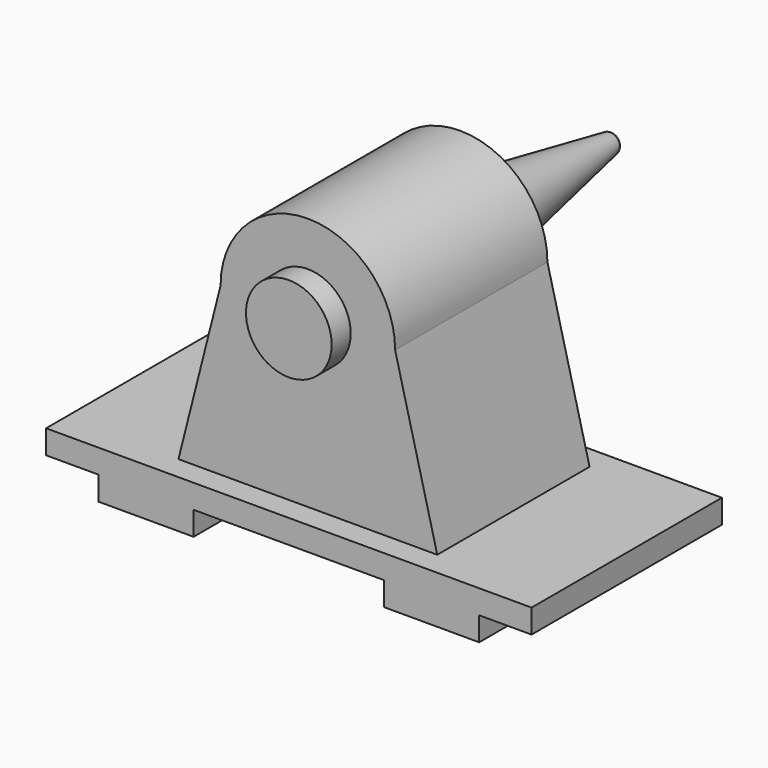
from build123d import *

# Parameters (mm, degrees)
F0_W      = 20
F0_H      = 5
F1_DEPTH  = 50
F2_START  = -5
F0_R      = 9
F2_DEPTH  = 40
F3_DEPTH  = 45
F3_FACE_R = 9
F4_DEPTH  = 40
F4_TAPER  = 10
F5_R      = 1


with BuildPart() as f1:
    # F0 (on Front) → F1 (new body)
    with BuildSketch(Plane.XZ):
        Polygon((-8.3973156512, 120.4740846279), (2.6026843488, 120.4740846279), (22.6026843488, 120.4740846279), (62.6026843488, 120.4740846279), (82.6026843488, 120.4740846279), (93.6026843488, 120.4740846279), (93.6026843488, 125.4740846279), (69.7901826352, 125.4740846279), (15.4151860625, 125.4740846279), (-8.3973156512, 125.4740846279), align=None)
        with Locations((12.6026843488, 117.9740846279)):
            Rectangle(F0_W, F0_H)
        with Locations((72.6026843488, 117.9740846279)):
            Rectangle(F0_W, F0_H)
    extrude(amount=-F1_DEPTH)

    # F0 (on Front) → F2 (join)
    with BuildSketch(Plane.XZ.offset(F2_START)):
        with BuildLine():
            Line((24.2665670812, 160.4740846279), (15.4151860625, 125.4740846279))
            Line((15.4151860625, 125.4740846279), (69.7901826352, 125.4740846279))
            Line((69.7901826352, 125.4740846279), (60.9388016164, 160.4740846279))
            ThreePointArc((60.9388016164, 160.4740846279), (42.6026843488, 178.8102018955), (24.2665670812, 160.4740846279))
        make_face()
        with Locations((42.6026843488, 160.4740846279)):
            Circle(F0_R, mode=Mode.SUBTRACT)
    extrude(amount=-F2_DEPTH)


with BuildPart() as f3:
    # F0 (on Front) → F3 (new body, through all)
    with BuildSketch(Plane.XZ):
        with Locations((42.6026843488, 160.4740846279)):
            Circle(F0_R)
    extrude(amount=-F3_DEPTH)

    # F3_face (on face) → F4 (join)
    with BuildSketch(Plane(origin=(42.6026843488, 45, 160.4740846279), x_dir=(-1, 0, 0), z_dir=(0, 1, 0))):
        Circle(F3_FACE_R)
    extrude(amount=F4_DEPTH, taper=F4_TAPER)

    # F5
    f5_edges = [f3.edges().sort_by_distance(p)[0] for p in [
        (44.549605, 85, 160.474085),
    ]]
    fillet(f5_edges, radius=F5_R)


solid = Compound([f1.part, f3.part])
